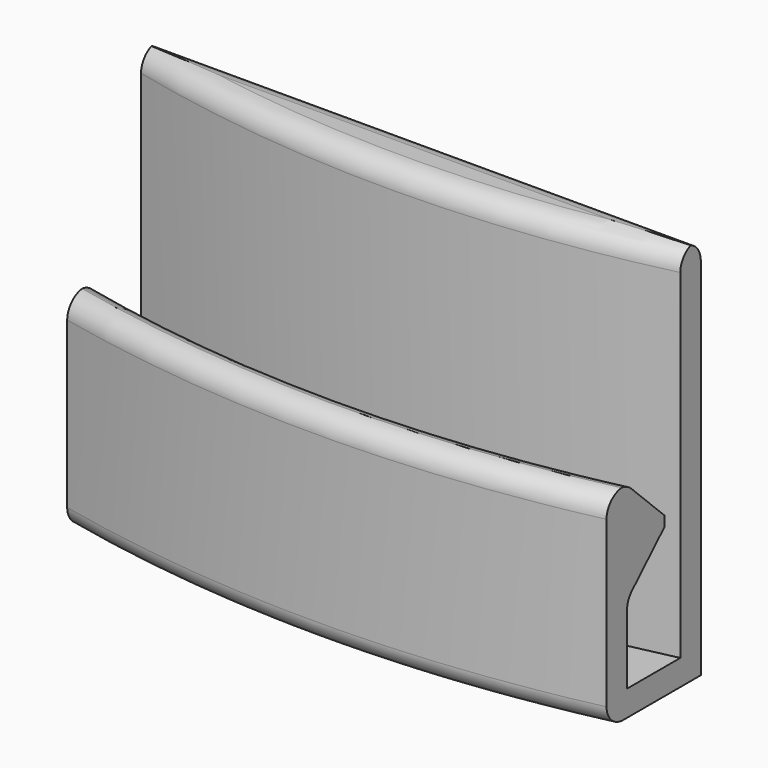
from build123d import *

# Parameters (mm, degrees)
F1_DEPTH      = 3.175
F3_DEPTH      = 22.225
F5_DEPTH      = 12.7
F6_T4_ANGLE   = 38.1311278428
F6_S5_R       = 150.8893647144
F6_T6_DEPTH   = 51
F6_T8_ANGLE   = 38.1311278428
F8_DEPTH      = 44.45
F10_DEPTH     = 66.675
F11_T4_ANGLE  = 27.5276640698
F11_T7_DEPTH  = 79.3798285845
F11_T10_ANGLE = 29.7338510625
F11_T12_ANGLE = 27.5124997685
F11_T14_ANGLE = 29.7338510625
F11_T16_ANGLE = 32.0818761549
F14_DEPTH     = 1.27


# Not quite as in the source:
# - a fillet or chamfer that OpenCascade refuses, or shapes differently, is made with other operations: its cross-section is extruded or revolved along the edge and cut away or added


with BuildPart() as f1:
    # F0 (on Top) → F1 (new body)
    with BuildSketch(Plane.XY):
        with BuildLine():
            Line((-15.875, -138.9311941889), (-17.4625, -138.9311941889))
            Line((-17.4625, -138.9311941889), (-26.9875, -138.9311941889))
            Line((-26.9875, -138.9311941889), (-33.3375, -138.9311941889))
            Line((-33.3375, -138.9311941889), (-33.3375, -150.3354956422))
            ThreePointArc((-33.3375, -150.3354956422), (0, -153.9875), (33.3375, -150.3354956422))
            Line((33.3375, -150.3354956422), (33.3375, -138.9311941889))
            Line((33.3375, -138.9311941889), (26.9875, -138.9311941889))
            Line((26.9875, -138.9311941889), (17.4625, -138.9311941889))
            Line((17.4625, -138.9311941889), (15.875, -138.9311941889))
            Line((15.875, -138.9311941889), (6.35, -138.9311941889))
            Line((6.35, -138.9311941889), (4.7625, -138.9311941889))
            Line((4.7625, -138.9311941889), (-4.7625, -138.9311941889))
            Line((-4.7625, -138.9311941889), (-6.35, -138.9311941889))
            Line((-6.35, -138.9311941889), (-15.875, -138.9311941889))
        make_face()
    extrude(amount=F1_DEPTH)

    # F2 (on face) → F3 (join)
    with BuildSketch(Plane.XY.offset(3.175)):
        with BuildLine():
            Line((-33.3375, -147.1604956422), (-33.3375, -150.3354956422))
            ThreePointArc((-33.3375, -150.3354956422), (0, -153.9875), (33.3375, -150.3354956422))
            Line((33.3375, -150.3354956422), (33.3375, -147.1604956422))
            ThreePointArc((33.3375, -147.1604956422), (0, -150.8893647144), (-33.3375, -147.1604956422))
        make_face()
    extrude(amount=F3_DEPTH)

    # F4 (on face) → F5 (join)
    with BuildSketch(Plane.XY.offset(25.4)):
        with BuildLine():
            Line((-33.3375, -141.3788854738), (-33.3375, -147.1604956422))
            ThreePointArc((-33.3375, -147.1604956422), (0, -150.8893647144), (33.3375, -147.1604956422))
            Line((33.3375, -147.1604956422), (33.3375, -141.3788854738))
            ThreePointArc((33.3375, -141.3788854738), (0, -145.25625), (-33.3375, -141.3788854738))
        make_face()
    extrude(amount=-F5_DEPTH)

    # F6: chamfer of 5.715 on 2 edges, made by hand


with BuildPart() as f6_tool2:
    # F6_s3 → F6_t4 (revolve)
    with BuildSketch(Plane(origin=(0, 0, 0), x_dir=(0, 0, 1), z_dir=(0.9451454069, 0.3266499039, 0))):
        Polygon((12.7, 150.97125), (18.415, 145.25625), (12.7, 145.25625), align=None)
    revolve(axis=Axis((0, 0, 12.7), (0, 0, -1)), revolution_arc=F6_T4_ANGLE)

    # F6_s5 → F6_t6 (intersect, symmetric)
    with BuildSketch(Plane.XY.offset(15.6)):
        Circle(F6_S5_R)
    extrude(amount=F6_T6_DEPTH, both=True, mode=Mode.INTERSECT)


with BuildPart() as f1_1:
    add(f1.part)

    # F6_t1: cut F6_tool2
    add(f6_tool2.part, mode=Mode.SUBTRACT)

    # F6_s7 → F6_t8 (revolve, cut)
    with BuildSketch(Plane(origin=(0, 0, 0), x_dir=(0, 0, 1), z_dir=(0.9451454069, 0.3266499039, 0))):
        Polygon((19.685, 145.25625), (25.4, 150.97125), (25.4, 145.25625), align=None)
    revolve(axis=Axis((0, 0, 25.4), (0, 0, -1)), revolution_arc=F6_T8_ANGLE, mode=Mode.SUBTRACT)

    # F7 (on face) → F8 (join)
    with BuildSketch(Plane.XY.offset(3.175)):
        with BuildLine():
            Line((33.3375, -138.9311941889), (-33.3375, -138.9311941889))
            ThreePointArc((-33.3375, -138.9311941889), (0, -142.875), (33.3375, -138.9311941889))
        make_face()
    extrude(amount=F8_DEPTH)

    # F9 (on face) → F10 (join, through all)
    with BuildSketch(Plane.YZ.offset(33.3375)):
        Polygon((-138.9311941889, 47.625), (-138.9311941889, 15.875), (-135.7561941889, 19.05), (-135.7561941889, 47.625), align=None)
    extrude(amount=-F10_DEPTH)

    # F11: fillet of radius 2.54 on 6 edges, made by hand


with BuildPart() as f11_tool2:
    # F11_s3 → F11_t4 (revolve)
    with BuildSketch(Plane(origin=(-1.5e-08, 3.7e-09, 0), x_dir=(0, 0, 1), z_dir=(-0.9712846607, 0.2379203815, 0))):
        with BuildLine():
            ThreePointArc((11.72895441, -150.8897647166), (12.7018887685, -150.69623604), (13.5267026905, -150.1451129971))
            Line((13.5267026905, -150.1451129971), (13.7064775186, -150.3248878251))
            ThreePointArc((13.7064775186, -150.3248878251), (13.3339273944, -150.6968722638), (12.9616601136, -151.0691395459))
            Line((12.9616601136, -151.0691395459), (12.7818852856, -151.1436047179))
            ThreePointArc((12.7818852856, -151.1436047179), (12.2554198478, -151.1436047166), (11.72895441, -151.1440047166))
            Line((11.72895441, -151.1440047166), (11.72895441, -150.8897647166))
        make_face()
    revolve(axis=Axis((-2.6e-09, 5.44e-08, 12.7818852856), (0, 0, 1)), revolution_arc=F11_T4_ANGLE)

    split(bisect_by=Plane.YZ.offset(33.3375), keep=Keep.BOTTOM)

    split(bisect_by=Plane.YZ.offset(-33.3375), keep=Keep.TOP)


with BuildPart() as f1_2:
    add(f1_1.part)

    # F11_t1: union F11_tool2
    add(f11_tool2.part)

    # F11_s8 → F11_t7 (cut)
    with BuildSketch(Plane.YZ.offset(-39.6899142923)):
        with BuildLine():
            ThreePointArc((-138.2971598743, 47.6254), (-136.5001429647, 46.8810512242), (-135.7557941889, 45.0840343146))
            Line((-135.7557941889, 45.0840343146), (-135.5016576203, 45.0840343146))
            ThreePointArc((-135.5016576203, 45.0840343146), (-135.5020576203, 46.3545171573), (-135.5020576203, 47.625))
            Line((-135.5020576203, 47.625), (-135.7561941889, 47.8791365685))
            ThreePointArc((-135.7561941889, 47.8791365685), (-137.0266770316, 47.8791365685), (-138.2971598743, 47.8795365685))
            Line((-138.2971598743, 47.8795365685), (-138.2971598743, 47.6254))
        make_face()
    extrude(amount=F11_T7_DEPTH, mode=Mode.SUBTRACT)

    # F11_s9 → F11_t10 (revolve, cut)
    with BuildSketch(Plane(origin=(0, 0, 0), x_dir=(0, 0, 1), z_dir=(-0.9665243504, 0.2565749017, 0))):
        with BuildLine():
            ThreePointArc((2.5409656854, -153.9879), (0.7439487758, -153.2435512242), (-0.0004, -151.4465343146))
            Line((-0.0004, -151.4465343146), (-0.2545365685, -151.4465343146))
            ThreePointArc((-0.2545365685, -151.4465343146), (-0.2541365685, -152.7170171573), (-0.2541365685, -153.9875))
            Line((-0.2541365685, -153.9875), (0, -154.2416365685))
            ThreePointArc((0, -154.2416365685), (1.2704828427, -154.2416365685), (2.5409656854, -154.2420365685))
            Line((2.5409656854, -154.2420365685), (2.5409656854, -153.9879))
        make_face()
    revolve(axis=Axis((0, 0, 0), (0, 0, 1)), revolution_arc=F11_T10_ANGLE, mode=Mode.SUBTRACT)

    # F11_s11 → F11_t12 (revolve, cut)
    with BuildSketch(Plane(origin=(0, 0, 0), x_dir=(0, 0, 1), z_dir=(0.971316137, 0.2377918459, 0))):
        with BuildLine():
            ThreePointArc((24.6557482805, 150.2264325951), (25.2068713235, 151.0512465171), (25.4004, 152.0241808756))
            Line((25.4004, 152.0241808756), (25.65464, 152.0241808756))
            ThreePointArc((25.65464, 152.0241808756), (25.65424, 151.4977154378), (25.65424, 150.97125))
            Line((25.65424, 150.97125), (25.579774828, 150.791475172))
            ThreePointArc((25.579774828, 150.791475172), (25.2075075469, 150.4192078908), (24.8355231085, 150.046657767))
            Line((24.8355231085, 150.046657767), (24.6557482805, 150.2264325951))
        make_face()
    revolve(axis=Axis((0, 0, 25.4), (0, 0, -1)), revolution_arc=F11_T12_ANGLE, mode=Mode.SUBTRACT)

    # F11_s13 → F11_t14 (revolve, cut)
    with BuildSketch(Plane(origin=(0, 0, 0), x_dir=(0, 0, 1), z_dir=(-0.9665243504, 0.2565749017, 0))):
        with BuildLine():
            ThreePointArc((22.8590343146, -153.9879), (24.6560512242, -153.2435512242), (25.4004, -151.4465343146))
            Line((25.4004, -151.4465343146), (25.6545365685, -151.4465343146))
            ThreePointArc((25.6545365685, -151.4465343146), (25.6541365685, -152.7170171573), (25.6541365685, -153.9875))
            Line((25.6541365685, -153.9875), (25.4, -154.2416365685))
            ThreePointArc((25.4, -154.2416365685), (24.1295171573, -154.2416365685), (22.8590343146, -154.2420365685))
            Line((22.8590343146, -154.2420365685), (22.8590343146, -153.9879))
        make_face()
    revolve(axis=Axis((0, 0, 25.4), (0, 0, 1)), revolution_arc=F11_T14_ANGLE, mode=Mode.SUBTRACT)

    # F11_s15 → F11_t16 (revolve, cut)
    with BuildSketch(Plane(origin=(0, 0, 0), x_dir=(0, 0, 1), z_dir=(-0.9610645065, 0.276324111, 0))):
        with BuildLine():
            ThreePointArc((45.0840343146, -142.8754), (46.8810512242, -142.1310512242), (47.6254, -140.3340343146))
            Line((47.6254, -140.3340343146), (47.8795365685, -140.3340343146))
            ThreePointArc((47.8795365685, -140.3340343146), (47.8791365685, -141.6045171573), (47.8791365685, -142.875))
            Line((47.8791365685, -142.875), (47.625, -143.1291365685))
            ThreePointArc((47.625, -143.1291365685), (46.3545171573, -143.1291365685), (45.0840343146, -143.1295365685))
            Line((45.0840343146, -143.1295365685), (45.0840343146, -142.8754))
        make_face()
    revolve(axis=Axis((0, 0, 47.625), (0, 0, 1)), revolution_arc=F11_T16_ANGLE, mode=Mode.SUBTRACT)

    # F13 (on face) → F14 (cut)
    with BuildSketch(Plane(origin=(0, -138.9311941889, 0), x_dir=(-1, 0, 0), z_dir=(0, 1, 0))):
        with BuildLine():
            Line((-26.9875, 44.45), (-26.9875, 15.875))
            Line((-26.9875, 15.875), (-17.4625, 15.875))
            Line((-17.4625, 15.875), (-17.4625, 44.45))
            Line((-17.4625, 44.45), (-18.923, 44.45))
            Line((-18.923, 44.45), (-18.923, 41.148))
            ThreePointArc((-18.923, 41.148), (-22.225, 37.846), (-25.527, 41.148))
            Line((-25.527, 41.148), (-25.527, 44.45))
            Line((-25.527, 44.45), (-26.9875, 44.45))
        make_face()
        with BuildLine():
            Line((-15.875, 44.45), (-15.875, 15.875))
            Line((-15.875, 15.875), (-6.35, 15.875))
            Line((-6.35, 15.875), (-6.35, 44.45))
            Line((-6.35, 44.45), (-7.8105, 44.45))
            Line((-7.8105, 44.45), (-7.8105, 41.148))
            ThreePointArc((-7.8105, 41.148), (-11.1125, 37.846), (-14.4145, 41.148))
            Line((-14.4145, 41.148), (-14.4145, 44.45))
            Line((-14.4145, 44.45), (-15.875, 44.45))
        make_face()
        with BuildLine():
            Line((-4.7625, 44.45), (-4.7625, 15.875))
            Line((-4.7625, 15.875), (4.7625, 15.875))
            Line((4.7625, 15.875), (4.7625, 44.45))
            Line((4.7625, 44.45), (3.302, 44.45))
            Line((3.302, 44.45), (3.302, 41.148))
            ThreePointArc((3.302, 41.148), (0, 37.846), (-3.302, 41.148))
            Line((-3.302, 41.148), (-3.302, 44.45))
            Line((-3.302, 44.45), (-4.7625, 44.45))
        make_face()
        with BuildLine():
            Line((6.35, 44.45), (6.35, 15.875))
            Line((6.35, 15.875), (15.875, 15.875))
            Line((15.875, 15.875), (15.875, 44.45))
            Line((15.875, 44.45), (14.4145, 44.45))
            Line((14.4145, 44.45), (14.4145, 41.148))
            ThreePointArc((14.4145, 41.148), (11.1125, 37.846), (7.8105, 41.148))
            Line((7.8105, 41.148), (7.8105, 44.45))
            Line((7.8105, 44.45), (6.35, 44.45))
        make_face()
        with BuildLine():
            Line((17.4625, 44.45), (17.4625, 15.875))
            Line((17.4625, 15.875), (26.9875, 15.875))
            Line((26.9875, 15.875), (26.9875, 44.45))
            Line((26.9875, 44.45), (25.527, 44.45))
            Line((25.527, 44.45), (25.527, 41.148))
            ThreePointArc((25.527, 41.148), (22.225, 37.846), (18.923, 41.148))
            Line((18.923, 41.148), (18.923, 44.45))
            Line((18.923, 44.45), (17.4625, 44.45))
        make_face()
    extrude(amount=F14_DEPTH, mode=Mode.SUBTRACT)

    # F15 (on face) → F16 (join, up to the next surface of F1)
    with BuildSketch(Plane(origin=(0, 0, 0), x_dir=(1, 0, 0), z_dir=(0, 0, -1))):
        with BuildLine():
            Line((-26.9875, 138.9311941889), (-33.3375, 138.9311941889))
            Line((-33.3375, 138.9311941889), (-33.3375, 135.7561941889))
            Line((-33.3375, 135.7561941889), (-30.1625, 135.7561941889))
            ThreePointArc((-30.1625, 135.7561941889), (-27.9174359697, 136.6861301586), (-26.9875, 138.9311941889))
        make_face()
        with BuildLine():
            Line((30.1625, 135.7561941889), (33.3375, 135.7561941889))
            Line((33.3375, 135.7561941889), (33.3375, 138.9311941889))
            Line((33.3375, 138.9311941889), (26.9875, 138.9311941889))
            ThreePointArc((26.9875, 138.9311941889), (27.9174359697, 136.6861301586), (30.1625, 135.7561941889))
        make_face()
    extrude(until=Until.NEXT, dir=(0, 0, 1))


solid = f1_2.part
